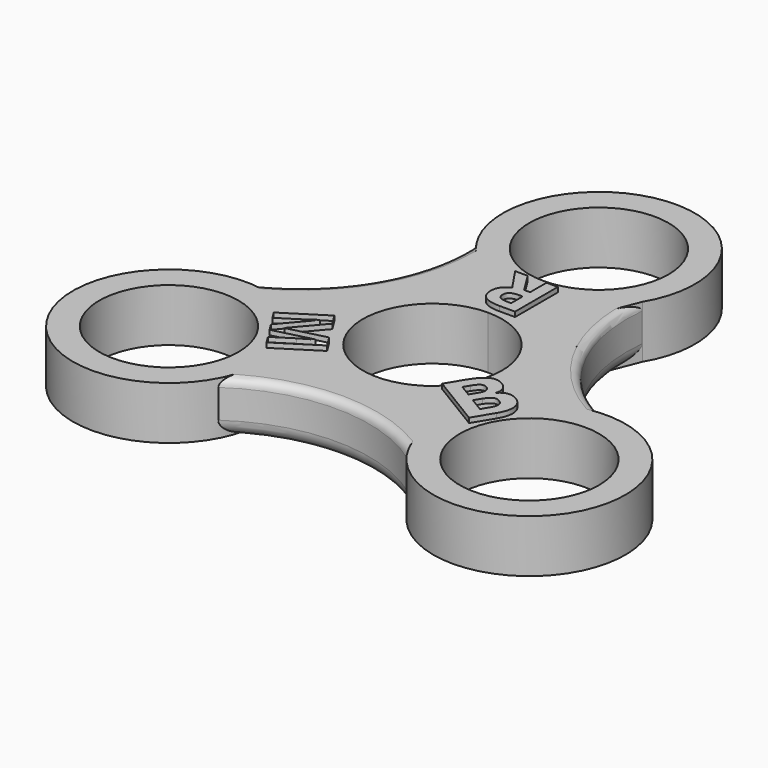
from build123d import *

# Parameters (mm, degrees)
F0_R           = 11.049
F1_DEPTH       = 8.382
F2_TEXT_SIZE   = 10.5833333333
F2_TEXT_SIZE_2 = 13.6077268204
F2_TEXT_SIZE_3 = 11.8899404899
F3_DEPTH       = 0.762
F4_R           = 1.27
F5_R           = 2.54


# Not quite as in the source:
# - Text() gives the source's letters only with a copy of the font that has no kerning and outlines rounded to 1/6400 em; it was checked with that copy


with BuildPart() as f1:
    # F0 (on Top) → F1 (new body)
    with BuildSketch(Plane.XY):
        with BuildLine():
            Line((13.0984179312, 25.2228158776), (13.1065708983, 25.2434069614))
            ThreePointArc((13.1065708983, 25.2434069614), (-0.2195384125, 48.2584186478), (-12.8771045205, 24.8690626817))
            ThreePointArc((-12.8771045205, 24.8690626817), (-16.4534691457, 9.3297508356), (-28.3748706399, -1.2599036912))
            ThreePointArc((-28.3748706399, -1.2599036912), (-41.6942634529, -24.2843876536), (-15.1038344264, -23.5900024393))
            ThreePointArc((-15.1038344264, -23.5900024393), (0.1536091548, -18.9140769793), (15.2943903394, -23.9549706166))
            ThreePointArc((15.2943903394, -23.9549706166), (41.893580025, -23.9317358457), (27.9589214054, -1.2746680535))
            ThreePointArc((27.9589214054, -1.2746680535), (16.2971690421, 9.6009342615), (13.0984179312, 25.2228158776))
        make_face()
        with Locations((-28.596158833, -16.51)):
            Circle(F0_R, mode=Mode.SUBTRACT)
        with Locations((28.596158833, -16.51)):
            Circle(F0_R, mode=Mode.SUBTRACT)
        with BuildLine():
            ThreePointArc((0, 11.049), (7.8128228253, 7.8128228253), (11.049, 0))
            ThreePointArc((11.049, 0), (-7.8128228253, -7.8128228253), (0, 11.049))
        make_face(mode=Mode.SUBTRACT)
        with BuildLine():
            ThreePointArc((11.049, 33.02), (7.8128228253, 25.2071771747), (0, 21.971))
            ThreePointArc((0, 21.971), (-7.8128228253, 40.8328228253), (11.049, 33.02))
        make_face(mode=Mode.SUBTRACT)
    extrude(amount=F1_DEPTH)

    # F2 (on face) → F3 (join)
    with BuildSketch(Plane.XY.offset(8.382)):
        with Locations(Location((-20.3611063585, -5.8573303649), (0, 0, -57.6498659638))):
            Text('M', F2_TEXT_SIZE, font='Open Sans', font_style=FontStyle.BOLD, text_align=(TextAlign.LEFT, TextAlign.BOTTOM))
        with Locations(Location((16.0346800312, -14.622946908), (0, 0, 58.7342887838))):
            Text('B', F2_TEXT_SIZE_2, font='Open Sans', font_style=FontStyle.BOLD, text_align=(TextAlign.LEFT, TextAlign.BOTTOM))
        with Locations(Location((4.4220844348, 20.6879815087), (0, 0, 180))):
            Text('R', F2_TEXT_SIZE_3, font='Open Sans', font_style=FontStyle.BOLD, text_align=(TextAlign.LEFT, TextAlign.BOTTOM))
    extrude(amount=F3_DEPTH)

    # F4
    f4_edges = [f1.edges().sort_by_distance(p)[0] for p in [
        (0.153609, -18.914077, 8.382),
        (16.297169, 9.600934, 8.382),
        (-16.453469, 9.329751, 8.382),
    ]]
    fillet(f4_edges, radius=F4_R)

    # F5
    f5_edges = [f1.edges().sort_by_distance(p)[0] for p in [
        (-16.453469, 9.329751, 0),
        (0.153609, -18.914077, 0),
        (16.297169, 9.600934, 0),
    ]]
    fillet(f5_edges, radius=F5_R)


solid = f1.part
